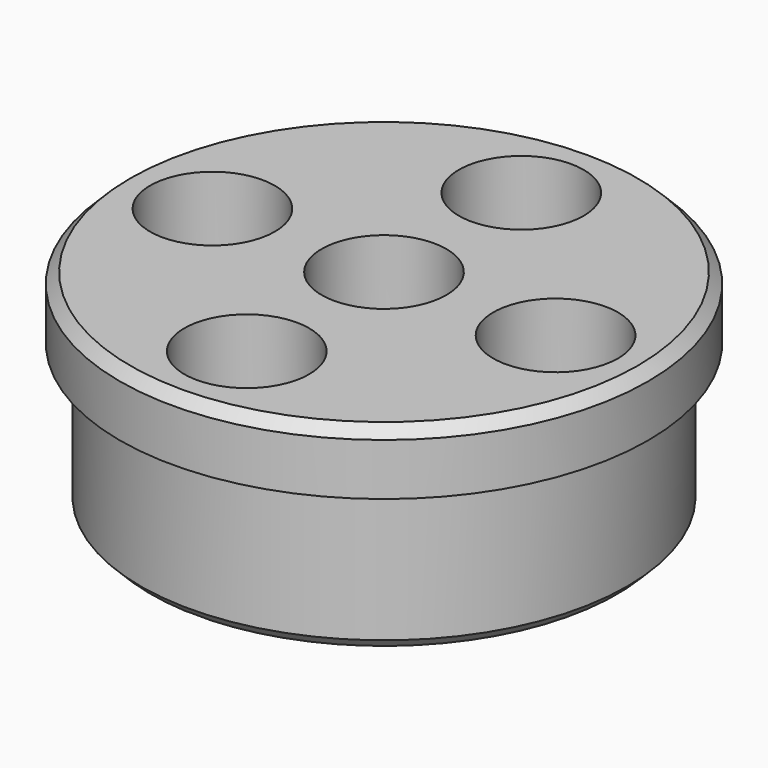
from build123d import *

# Parameters (mm, degrees)
F0_R     = 12.7
F0_R_2   = 3
F1_DEPTH = 10
F2_R     = 12.7
F2_R_2   = 11.7
F3_DEPTH = 7


# Not quite as in the source:
# - a fillet or chamfer that OpenCascade refuses, or shapes differently, is made with other operations: its cross-section is extruded or revolved along the edge and cut away or added


with BuildPart() as f1:
    # F0 (on Top) → F1 (new body)
    with BuildSketch(Plane.XY):
        with Locations((0.256980346, -0.0691873614)):
            Circle(F0_R)
        with Locations((0.256980346, -8.3191873614)):
            Circle(F0_R_2, mode=Mode.SUBTRACT)
        with Locations((-7.993019654, -0.0691873614)):
            Circle(F0_R_2, mode=Mode.SUBTRACT)
        with Locations((0.256980346, -0.0691873614)):
            Circle(F0_R_2, mode=Mode.SUBTRACT)
        with Locations((8.506980346, -0.0691873614)):
            Circle(F0_R_2, mode=Mode.SUBTRACT)
        with Locations((0.256980346, 8.1808126386)):
            Circle(F0_R_2, mode=Mode.SUBTRACT)
    extrude(amount=F1_DEPTH)

    # F2 (on face) → F3 (cut)
    with BuildSketch(Plane(origin=(0, 0, 0), x_dir=(1, 0, 0), z_dir=(0, 0, -1))):
        with Locations((0.256980346, 0.0691873614)):
            Circle(F2_R)
        with Locations((0.256980346, 0.0691873614)):
            Circle(F2_R_2, mode=Mode.SUBTRACT)
    extrude(amount=-F3_DEPTH, mode=Mode.SUBTRACT)

    # F4: chamfer of 0.5 on 2 edges, made by hand

    # F4_s1 → F4_t2 (revolve, cut)
    with BuildSketch(Plane.XZ.offset(0.0691873614)):
        Polygon((12.956980346, 9.5), (12.456980346, 10), (12.956980346, 10), align=None)
    revolve(axis=Axis((0.256980346, -0.0691873614, 10), (0, 0, 1)), mode=Mode.SUBTRACT)

    # F4_s3 → F4_t4 (revolve, cut)
    with BuildSketch(Plane.XZ.offset(0.0691873614)):
        Polygon((11.956980346, 0.5), (11.456980346, 0), (11.956980346, 0), align=None)
    revolve(axis=Axis((0.256980346, -0.0691873614, 0), (0, 0, -1)), mode=Mode.SUBTRACT)


solid = f1.part
